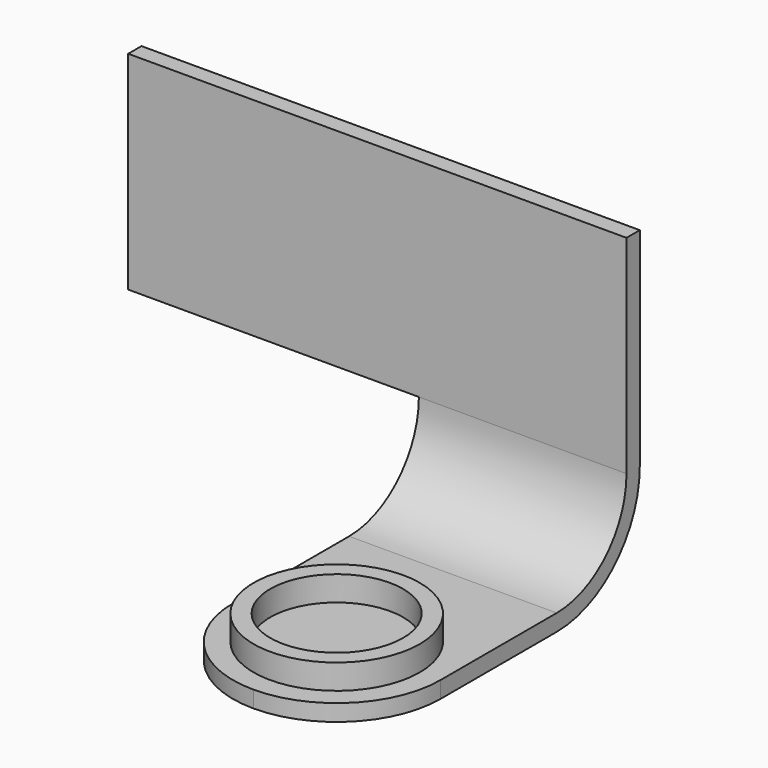
from build123d import *

# Parameters (mm, degrees)
F0_W     = 60
F0_H     = 25
F1_DEPTH = 2
F3_DEPTH = 12.5
F4_R     = 12.49999
F5_R     = 10
F5_R_2   = 8
F6_DEPTH = 3


# Not quite as in the source:
# - a fillet or chamfer is up to 0.001 mm smaller than in the source, because OpenCascade refuses the exact size


with BuildPart() as f1:
    # F0 (on Front) → F1 (new body)
    with BuildSketch(Plane.XZ):
        with Locations((-17.5, 12.5)):
            Rectangle(F0_W, F0_H)
    extrude(amount=F1_DEPTH)

    # F2 (on Right) → F3 (join, symmetric)
    with BuildSketch(Plane.YZ):
        with BuildLine():
            Line((-42.5, -12.5), (-12.5, -12.5))
            ThreePointArc((-12.5, -12.5), (-3.6611652352, -8.8388347648), (0, 0))
            Line((0, 0), (-2, 0))
            ThreePointArc((-2, 0), (-5.0753787975, -7.4246212025), (-12.5, -10.5))
            Line((-12.5, -10.5), (-42.5, -10.5))
            Line((-42.5, -10.5), (-42.5, -12.5))
        make_face()
    extrude(amount=F3_DEPTH, both=True)

    # F4 (radius 12.5 in the source; OpenCascade refuses exactly that, so slightly less here)
    f4_edges = [f1.edges().sort_by_distance(p)[0] for p in [
        (-12.5, -42.5, -11.5),
        (12.5, -42.5, -11.5),
    ]]
    fillet(f4_edges, radius=F4_R)

    # F5 (on face) → F6 (join)
    with BuildSketch(Plane.XY.offset(-10.5)):
        with Locations((0, -30)):
            Circle(F5_R)
        with Locations((0, -30)):
            Circle(F5_R_2, mode=Mode.SUBTRACT)
    extrude(amount=F6_DEPTH)


solid = f1.part
